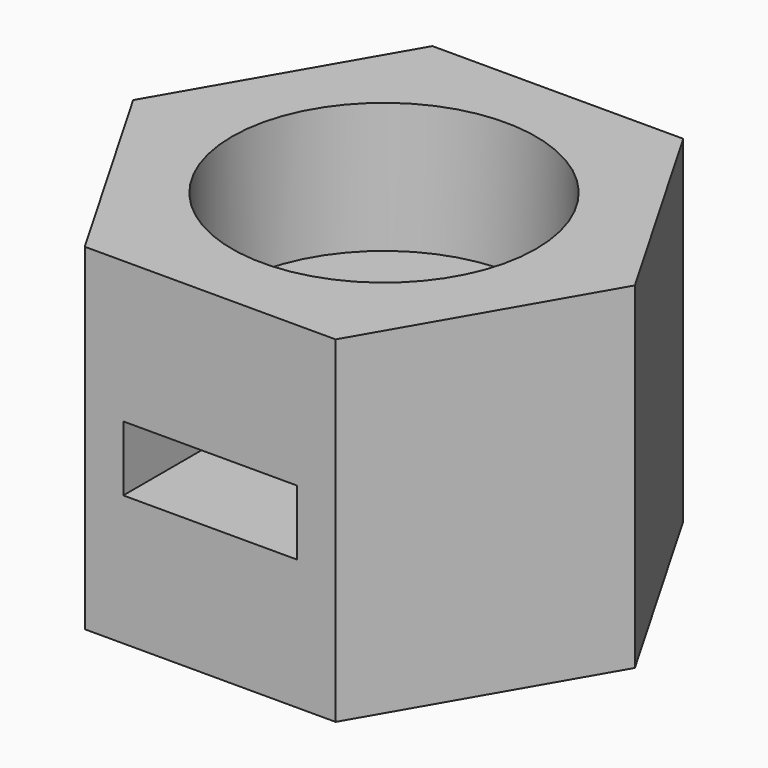
from build123d import *

# Parameters (mm, degrees)
F1_DEPTH = 12.065
F2_W     = 10.16
F2_H     = 3.81
F3_DEPTH = 25.4010101543
F5_W     = 13.97
F5_H     = 5.08
F6_DEPTH = 8.255
F4_R     = 8.89
F7_DEPTH = 7.62
F8_R     = 9.525
F9_DEPTH = 2.54


# Not quite as in the source:
# - a feature names something its author has since deleted; it is built from what else it names


with BuildPart() as f1:
    # F0 (on Top) → F1 (new body)
    with BuildSketch(Plane.XY):
        Polygon((7.33235135, -12.7000050771), (14.6647027, 0), (7.33235135, 12.7000050771), (-7.33235135, 12.7000050771), (-14.6647027, 0), (-7.33235135, -12.7000050771), align=None)
    extrude(amount=F1_DEPTH)

    # F2 (on face) → F3 (cut, through all)
    with BuildSketch(Plane.XZ.offset(12.7000050771)):
        with Locations((0, 9.525)):
            Rectangle(F2_W, F2_H)
    extrude(amount=-F3_DEPTH, mode=Mode.SUBTRACT)

    # F5 (on face) → F6 (cut)
    with BuildSketch(Plane.XY.offset(12.065)):
        Rectangle(F5_W, F5_H)
    extrude(amount=-F6_DEPTH, mode=Mode.SUBTRACT)

    # F4 (on face) → F7 (join)
    with BuildSketch(Plane.XY.offset(12.065)):
        Polygon((-7.33235135, -12.7000050771), (7.33235135, -12.7000050771), (14.6647027, 0), (7.33235135, 12.7000050771), (-7.33235135, 12.7000050771), (-14.6647027, 0), align=None)
        Circle(F4_R, mode=Mode.SUBTRACT)
    extrude(amount=F7_DEPTH)

    # F8 (on face) → F9 (cut)
    with BuildSketch(Plane(origin=(0, 0, 0), x_dir=(1, 0, 0), z_dir=(0, 0, -1))):
        Circle(F8_R)
    extrude(amount=-F9_DEPTH, mode=Mode.SUBTRACT)


solid = f1.part
